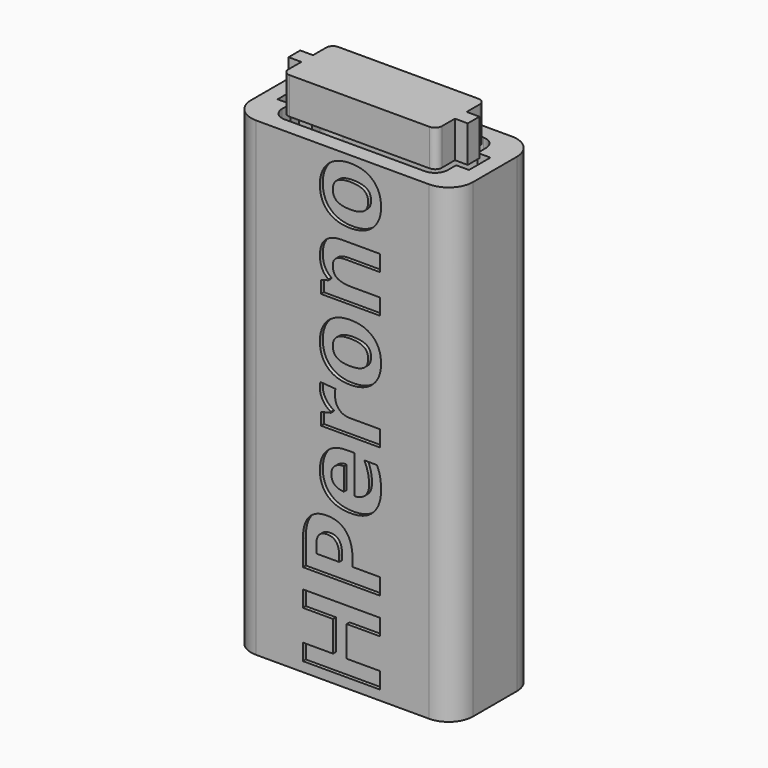
from build123d import *

# Parameters (mm, degrees)
F1_DEPTH     = 36.6
F0_W         = 0.7
F0_H         = 0.3
F0_W_2       = 0.25
F2_DEPTH     = 2
F3_TEXT_SIZE = 8.8665566004
F4_DEPTH     = 0.3
F5_W         = 1.05
F5_H         = 1.2
F6_DEPTH     = 3


# Not quite as in the source:
# - Text() gives the source's letters only with a copy of the font that has no kerning and outlines rounded to 1/6400 em; it was checked with that copy


with BuildPart() as f1:
    # F0 (on Top) → F1 (new body)
    with BuildSketch(Plane.XY):
        with BuildLine():
            ThreePointArc((-9.1, -2.35), (-8.5142135624, -3.7642135624), (-7.1, -4.35))
            Line((-7.1, -4.35), (7.1, -4.35))
            ThreePointArc((7.1, -4.35), (8.5142135624, -3.7642135624), (9.1, -2.35))
            Line((9.1, -2.35), (9.1, 2.15))
            ThreePointArc((9.1, 2.15), (8.5142135624, 3.5642135624), (7.1, 4.15))
            Line((7.1, 4.15), (-7.1, 4.15))
            ThreePointArc((-7.1, 4.15), (-8.5142135624, 3.5642135624), (-9.1, 2.15))
            Line((-9.1, 2.15), (-9.1, -2.35))
        make_face()
        with BuildLine():
            Line((-7.85, 1), (-6.8, 1))
            Line((-6.8, 1), (-6.8, 1.85))
            ThreePointArc((-6.8, 1.85), (-6.4924621202, 2.5924621202), (-5.75, 2.9))
            Line((-5.75, 2.9), (5.75, 2.9))
            ThreePointArc((5.75, 2.9), (6.4924621202, 2.5924621202), (6.8, 1.85))
            Line((6.8, 1.85), (6.8, 1))
            Line((6.8, 1), (7.85, 1))
            Line((7.85, 1), (7.85, 0))
            Line((7.85, 0), (7.85, -1.2))
            Line((7.85, -1.2), (6.8, -1.2))
            Line((6.8, -1.2), (6.8, -2.05))
            ThreePointArc((6.8, -2.05), (6.4924621202, -2.7924621202), (5.75, -3.1))
            Line((5.75, -3.1), (-5.75, -3.1))
            ThreePointArc((-5.75, -3.1), (-6.4924621202, -2.7924621202), (-6.8, -2.05))
            Line((-6.8, -2.05), (-6.8, -1.2))
            Line((-6.8, -1.2), (-7.85, -1.2))
            Line((-7.85, -1.2), (-7.85, 0))
            Line((-7.85, 0), (-7.85, 1))
        make_face(mode=Mode.SUBTRACT)
    extrude(amount=F1_DEPTH)

    # F0 (on Top) → F2 (join)
    with BuildSketch(Plane.XY):
        with BuildLine():
            ThreePointArc((-9.1, -2.35), (-8.5142135624, -3.7642135624), (-7.1, -4.35))
            Line((-7.1, -4.35), (7.1, -4.35))
            ThreePointArc((7.1, -4.35), (8.5142135624, -3.7642135624), (9.1, -2.35))
            Line((9.1, -2.35), (9.1, 2.15))
            ThreePointArc((9.1, 2.15), (8.5142135624, 3.5642135624), (7.1, 4.15))
            Line((7.1, 4.15), (-7.1, 4.15))
            ThreePointArc((-7.1, 4.15), (-8.5142135624, 3.5642135624), (-9.1, 2.15))
            Line((-9.1, 2.15), (-9.1, -2.35))
        make_face()
        with BuildLine():
            Line((-7.85, 1), (-6.8, 1))
            Line((-6.8, 1), (-6.8, 1.85))
            ThreePointArc((-6.8, 1.85), (-6.4924621202, 2.5924621202), (-5.75, 2.9))
            Line((-5.75, 2.9), (5.75, 2.9))
            ThreePointArc((5.75, 2.9), (6.4924621202, 2.5924621202), (6.8, 1.85))
            Line((6.8, 1.85), (6.8, 1))
            Line((6.8, 1), (7.85, 1))
            Line((7.85, 1), (7.85, 0))
            Line((7.85, 0), (7.85, -1.2))
            Line((7.85, -1.2), (6.8, -1.2))
            Line((6.8, -1.2), (6.8, -2.05))
            ThreePointArc((6.8, -2.05), (6.4924621202, -2.7924621202), (5.75, -3.1))
            Line((5.75, -3.1), (-5.75, -3.1))
            ThreePointArc((-5.75, -3.1), (-6.4924621202, -2.7924621202), (-6.8, -2.05))
            Line((-6.8, -2.05), (-6.8, -1.2))
            Line((-6.8, -1.2), (-7.85, -1.2))
            Line((-7.85, -1.2), (-7.85, 0))
            Line((-7.85, 0), (-7.85, 1))
        make_face(mode=Mode.SUBTRACT)
        with BuildLine():
            Line((-6.1, -2.05), (-6.1, -0.4))
            Line((-6.1, -0.4), (-6.8, -0.4))
            Line((-6.8, -0.4), (-6.8, -1.2))
            Line((-6.8, -1.2), (-6.8, -2.05))
            ThreePointArc((-6.8, -2.05), (-6.4924621202, -2.7924621202), (-5.75, -3.1))
            Line((-5.75, -3.1), (5.75, -3.1))
            ThreePointArc((5.75, -3.1), (6.4924621202, -2.7924621202), (6.8, -2.05))
            Line((6.8, -2.05), (6.8, -1.2))
            Line((6.8, -1.2), (6.8, -0.4))
            Line((6.8, -0.4), (6.1, -0.4))
            Line((6.1, -0.4), (6.1, -2.05))
            ThreePointArc((6.1, -2.05), (5.9974873734, -2.2974873734), (5.75, -2.4))
            Line((5.75, -2.4), (-5.75, -2.4))
            ThreePointArc((-5.75, -2.4), (-5.9974873734, -2.2974873734), (-6.1, -2.05))
        make_face()
        with BuildLine():
            Line((-6.8, 0.2), (-6.1, 0.2))
            Line((-6.1, 0.2), (-6.1, 0.4))
            Line((-6.1, 0.4), (-6.1, 1.85))
            ThreePointArc((-6.1, 1.85), (-5.9974873734, 2.0974873734), (-5.75, 2.2))
            Line((-5.75, 2.2), (5.75, 2.2))
            ThreePointArc((5.75, 2.2), (5.9974873734, 2.0974873734), (6.1, 1.85))
            Line((6.1, 1.85), (6.1, 0.4))
            Line((6.1, 0.4), (6.1, 0.2))
            Line((6.1, 0.2), (6.8, 0.2))
            Line((6.8, 0.2), (6.8, 1))
            Line((6.8, 1), (6.8, 1.85))
            ThreePointArc((6.8, 1.85), (6.4924621202, 2.5924621202), (5.75, 2.9))
            Line((5.75, 2.9), (-5.75, 2.9))
            ThreePointArc((-5.75, 2.9), (-6.4924621202, 2.5924621202), (-6.8, 1.85))
            Line((-6.8, 1.85), (-6.8, 1))
            Line((-6.8, 1), (-6.8, 0.2))
        make_face()
        Polygon((-7.05, 0.2), (-6.8, 0.2), (-6.8, 1), (-7.85, 1), (-7.85, 0), (-7.85, -1.2), (-6.8, -1.2), (-6.8, -0.4), (-7.05, -0.4), (-7.05, -0.1), align=None)
        Polygon((6.8, 1), (6.8, 0.2), (7.05, 0.2), (7.05, -0.1), (7.05, -0.4), (6.8, -0.4), (6.8, -1.2), (7.85, -1.2), (7.85, 0), (7.85, 1), align=None)
        with Locations((-6.45, -0.25)):
            Rectangle(F0_W, F0_H)
        with Locations((-6.45, 0.05)):
            Rectangle(F0_W, F0_H)
        with Locations((6.45, 0.05)):
            Rectangle(F0_W, F0_H)
        with Locations((6.45, -0.25)):
            Rectangle(F0_W, F0_H)
        with Locations((-6.925, 0.05)):
            Rectangle(F0_W_2, F0_H)
        with Locations((-6.925, -0.25)):
            Rectangle(F0_W_2, F0_H)
        with Locations((6.925, 0.05)):
            Rectangle(F0_W_2, F0_H)
        with Locations((6.925, -0.25)):
            Rectangle(F0_W_2, F0_H)
    extrude(amount=-F2_DEPTH)

    # F3 (on face) → F4 (cut)
    with BuildSketch(Plane.XZ.offset(4.35)):
        with Locations(Location((3.0718447347, -2), (0, 0, 90))):
            Text('HPerono', F3_TEXT_SIZE, font='Open Sans', font_style=FontStyle.BOLD, text_align=(TextAlign.LEFT, TextAlign.BOTTOM))
    extrude(amount=-F4_DEPTH, mode=Mode.SUBTRACT)


with BuildPart() as f6:
    # F5 (on face) → F6 (new body)
    with BuildSketch(Plane.XY.offset(36.6)):
        with Locations((6.825, -0.1)):
            Rectangle(F5_W, F5_H)
        with BuildLine():
            Line((6.3, -2.05), (6.3, -0.7))
            Line((6.3, -0.7), (6.3, 0.5))
            Line((6.3, 0.5), (6.3, 1.85))
            ThreePointArc((6.3, 1.85), (6.1389087297, 2.2389087297), (5.75, 2.4))
            Line((5.75, 2.4), (-5.75, 2.4))
            ThreePointArc((-5.75, 2.4), (-6.1389087297, 2.2389087297), (-6.3, 1.85))
            Line((-6.3, 1.85), (-6.3, 0.5))
            Line((-6.3, 0.5), (-6.3, -0.7))
            Line((-6.3, -0.7), (-6.3, -2.05))
            ThreePointArc((-6.3, -2.05), (-6.1389087297, -2.4389087297), (-5.75, -2.6))
            Line((-5.75, -2.6), (5.75, -2.6))
            ThreePointArc((5.75, -2.6), (6.1389087297, -2.4389087297), (6.3, -2.05))
        make_face()
        with Locations((-6.825, -0.1)):
            Rectangle(F5_W, F5_H)
    extrude(amount=F6_DEPTH)


solid = Compound([f1.part, f6.part])
